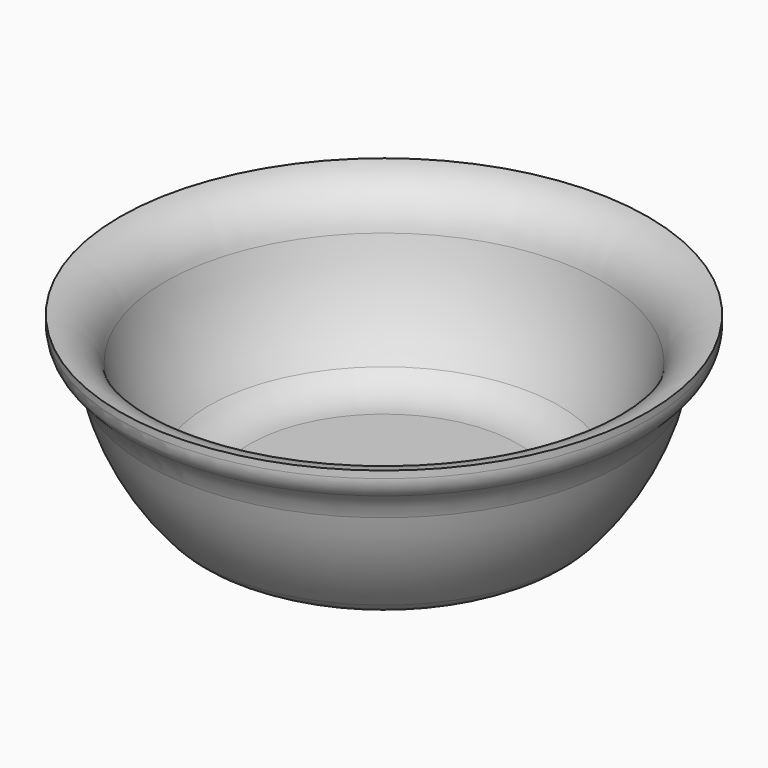
from build123d import *


# Not quite as in the source:
# - a fillet or chamfer that OpenCascade refuses, or shapes differently, is made with other operations: its cross-section is extruded or revolved along the edge and cut away or added


with BuildPart() as f1:
    # F0 (on Front) → F1 (revolve)
    with BuildSketch(Plane.XZ):
        with BuildLine():
            Line((0, -34), (0, -30))
            Line((0, -30), (-30, -30))
            ThreePointArc((-30, -30), (-39.1968889463, -16.2358830044), (-42.4264068712, 0))
            Line((-42.4264068712, 0), (-50.3107011318, 0))
            Line((-50.3107011318, 0), (-50.3107011318, -4))
            Line((-50.3107011318, -4), (-46.2537701703, -4))
            ThreePointArc((-46.2537701703, -4), (-41.7232145336, -20.361351231), (-31.6134663549, -34))
            Line((-31.6134663549, -34), (0, -34))
        make_face()
    revolve(axis=Axis((0, 0, -15), (0, 0, -1)))

    # F2: fillet of radius 10 on 4 edges, made by hand

    # F2_s1 → F2_t2 (revolve)
    with BuildSketch(Plane.XZ):
        with BuildLine():
            ThreePointArc((-25.5239468456, -30), (-29.9012676169, -28.9910546025), (-33.395292859, -26.1678125731))
            ThreePointArc((-33.395292859, -26.1678125731), (-31.7555066766, -28.135170085), (-30, -30))
            Line((-30, -30), (-25.5239468456, -30))
        make_face()
    revolve(axis=Axis((0, 0, -30), (0, 0, -1)))

    # F2_s3 → F2_t4 (revolve)
    with BuildSketch(Plane.XZ):
        with BuildLine():
            ThreePointArc((-45.2038898575, -10.5839310619), (-47.0388945384, -6.73473945), (-50.3107011318, -4))
            Line((-50.3107011318, -4), (-46.2537701703, -4))
            ThreePointArc((-46.2537701703, -4), (-45.8471692855, -7.310836031), (-45.2038898575, -10.5839310619))
        make_face()
    revolve(axis=Axis((0, 0, -4), (0, 0, -1)))

    # F2_s5 → F2_t6 (revolve, cut)
    with BuildSketch(Plane.XZ):
        with BuildLine():
            ThreePointArc((-50.3107011318, 0), (-44.671276634, -2.6050008536), (-41.6581484398, -8.0373296912))
            ThreePointArc((-41.6581484398, -8.0373296912), (-42.2339055452, -4.0369818424), (-42.4264068712, 0))
            Line((-42.4264068712, 0), (-50.3107011318, 0))
        make_face()
    revolve(axis=Axis((0, 0, 0), (0, 0, -1)), mode=Mode.SUBTRACT)

    # F2_s7 → F2_t8 (revolve, cut)
    with BuildSketch(Plane.XZ):
        with BuildLine():
            ThreePointArc((-34.9248789027, -30.5886267852), (-31.5322424712, -33.1073121131), (-27.4022465784, -34))
            Line((-27.4022465784, -34), (-31.6134663549, -34))
            ThreePointArc((-31.6134663549, -34), (-33.3128685977, -32.3367289744), (-34.9248789027, -30.5886267852))
        make_face()
    revolve(axis=Axis((0, 0, -34), (0, 0, -1)), mode=Mode.SUBTRACT)

    # F3: fillet of radius 5 on 2 edges, made by hand

    # F3_s1 → F3_t2 (revolve, cut)
    with BuildSketch(Plane.XZ):
        with BuildLine():
            ThreePointArc((-48.5206561627, -5.1965315899), (-49.8411412404, -3.478416904), (-50.3107011318, -1.3629707518))
            Line((-50.3107011318, -1.3629707518), (-50.3107011318, -4))
            ThreePointArc((-50.3107011318, -4), (-49.3833812624, -4.5499479973), (-48.5206561627, -5.1965315899))
        make_face()
    revolve(axis=Axis((0, 0, -4), (0, 0, -1)), mode=Mode.SUBTRACT)


solid = f1.part
